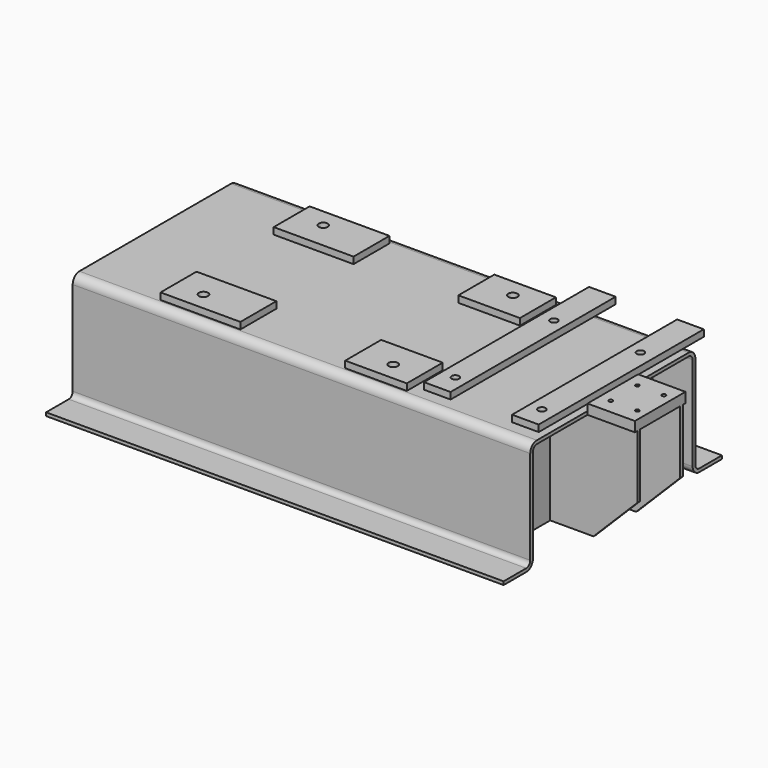
from build123d import *

# Parameters (mm, degrees)
F1_DEPTH  = 873.125
F4_DEPTH  = 12.7
F5_W      = 304.8
F5_H      = 171.45
F5_R      = 17.4625
F5_W_2    = 234.95
F6_DEPTH  = 25.4
F7_W      = 101.6
F7_H      = 787.4
F7_R      = 14.2875
F8_DEPTH  = 25.4
F9_W      = 180.848
F9_H      = 241.3
F10_DEPTH = 12.7
F12_W     = 333.248
F12_H     = 409.448
F13_DEPTH = 12.7
F14_SIZE  = 168.148
F16_R     = 7.14375
F17_DEPTH = 422.149
F18_W     = 180.848
F18_H     = 241.3
F18_R     = 7.324206161
F18_R_2   = 7.2547005792
F18_R_3   = 7.130511654
F18_R_4   = 7.4581094532
F19_DEPTH = 25.4


with BuildPart() as f1:
    # F0 (on Right) → F1 (new body, symmetric)
    with BuildSketch(Plane.YZ):
        with BuildLine():
            Line((361.95, 211.074), (-361.95, 211.074))
            ThreePointArc((-361.95, 211.074), (-384.4006403027, 201.7746403027), (-393.7, 179.324))
            Line((-393.7, 179.324), (-393.7, -179.324))
            ThreePointArc((-393.7, -179.324), (-399.2796158184, -192.7943841816), (-412.75, -198.374))
            Line((-412.75, -198.374), (-520.7, -198.374))
            Line((-520.7, -198.374), (-520.7, -211.074))
            Line((-520.7, -211.074), (-412.75, -211.074))
            ThreePointArc((-412.75, -211.074), (-390.2993596973, -201.7746403027), (-381, -179.324))
            Line((-381, -179.324), (-381, 179.324))
            ThreePointArc((-381, 179.324), (-375.4203841816, 192.7943841816), (-361.95, 198.374))
            Line((-361.95, 198.374), (361.95, 198.374))
            ThreePointArc((361.95, 198.374), (375.4203841816, 192.7943841816), (381, 179.324))
            Line((381, 179.324), (381, -179.324))
            ThreePointArc((381, -179.324), (390.2993596973, -201.7746403027), (412.75, -211.074))
            Line((412.75, -211.074), (520.7, -211.074))
            Line((520.7, -211.074), (520.7, -198.374))
            Line((520.7, -198.374), (412.75, -198.374))
            ThreePointArc((412.75, -198.374), (399.2796158184, -192.7943841816), (393.7, -179.324))
            Line((393.7, -179.324), (393.7, 179.324))
            ThreePointArc((393.7, 179.324), (384.4006403027, 201.7746403027), (361.95, 211.074))
        make_face()
    extrude(amount=F1_DEPTH, both=True)



with BuildPart() as f4:
    # F3 (on offset) → F4 (new body)
    with BuildSketch(Plane.YZ.offset(720.725)):
        Polygon((361.95, 198.374), (-361.95, 198.374), (-381, 179.324), (-381, -211.074), (381, -211.074), (381, 179.324), align=None)
    extrude(amount=-F4_DEPTH)


with BuildPart() as f1_1:
    add(f1.part)

    add(f4.part)  # F6 merges F4
    # F5 (on face) → F6 (join)
    with BuildSketch(Plane.XY.offset(211.074)):
        with Locations((-415.925, -269.875)):
            Rectangle(F5_W, F5_H)
        with Locations((-460.375, -285.75)):
            Circle(F5_R, mode=Mode.SUBTRACT)
        with Locations((254, -269.875)):
            Rectangle(F5_W_2, F5_H)
        with Locations((263.525, -285.75)):
            Circle(F5_R, mode=Mode.SUBTRACT)
        with Locations((-415.925, 269.875)):
            Rectangle(F5_W, F5_H)
        with Locations((-460.375, 285.75)):
            Circle(F5_R, mode=Mode.SUBTRACT)
        with Locations((254, 269.875)):
            Rectangle(F5_W_2, F5_H)
        with Locations((263.525, 285.75)):
            Circle(F5_R, mode=Mode.SUBTRACT)
    extrude(amount=F6_DEPTH)

    # F7 (on face) → F8 (join)
    with BuildSketch(Plane.XY.offset(211.074)):
        with Locations((457.327, 76.2)):
            Rectangle(F7_W, F7_H)
        with Locations((460.375, -234.95)):
            Circle(F7_R, mode=Mode.SUBTRACT)
        with Locations((460.375, 234.95)):
            Circle(F7_R, mode=Mode.SUBTRACT)
        with Locations((793.623, 76.2)):
            Rectangle(F7_W, F7_H)
        with Locations((790.575, -234.95)):
            Circle(F7_R, mode=Mode.SUBTRACT)
        with Locations((790.575, 234.95)):
            Circle(F7_R, mode=Mode.SUBTRACT)
    extrude(amount=F8_DEPTH)

    # F9 (on face) → F10 (join)
    with BuildSketch(Plane.XY.offset(211.074)):
        with Locations((963.549, 0)):
            Rectangle(F9_W, F9_H)
    extrude(amount=-F10_DEPTH)



with BuildPart() as f13:
    # F12 (on offset) → F13 (new body)
    with BuildSketch(Plane.XZ.offset(-95.25)):
        with Locations((887.349, -6.35)):
            Rectangle(F12_W, F12_H)
    extrude(amount=-F13_DEPTH)

    # F14
    f14_edges = [f13.edges().sort_by_distance(p)[0] for p in [
        (1053.973, 101.6, -211.074),
    ]]
    chamfer(f14_edges, length=F14_SIZE)


with BuildPart() as f1_2:
    add(f1_1.part)

    add(f13.part)  # F15 merges F13
    # F15: F13 across plane
    add(f13.part.mirror(Plane.XZ))

    # F16 (on face) → F17 (cut, through all)
    with BuildSketch(Plane.XY.offset(211.074)):
        with Locations((916.051, 63.5)):
            Circle(F16_R)
        with Locations((1017.651, 63.5)):
            Circle(F16_R)
        with Locations((1017.651, -63.5)):
            Circle(F16_R)
        with Locations((916.051, -63.5)):
            Circle(F16_R)
    extrude(amount=-F17_DEPTH, mode=Mode.SUBTRACT)

    # F18 (on face) → F19 (join)
    with BuildSketch(Plane.XY.offset(211.074)):
        with Locations((963.549, 0)):
            Rectangle(F18_W, F18_H)
        with Locations((916.051, -63.5)):
            Circle(F18_R, mode=Mode.SUBTRACT)
        with Locations((1017.651, -63.5)):
            Circle(F18_R_2, mode=Mode.SUBTRACT)
        with Locations((916.051, 63.5)):
            Circle(F18_R_3, mode=Mode.SUBTRACT)
        with Locations((1017.651, 63.5)):
            Circle(F18_R_4, mode=Mode.SUBTRACT)
    extrude(amount=F19_DEPTH)


solid = f1_2.part
